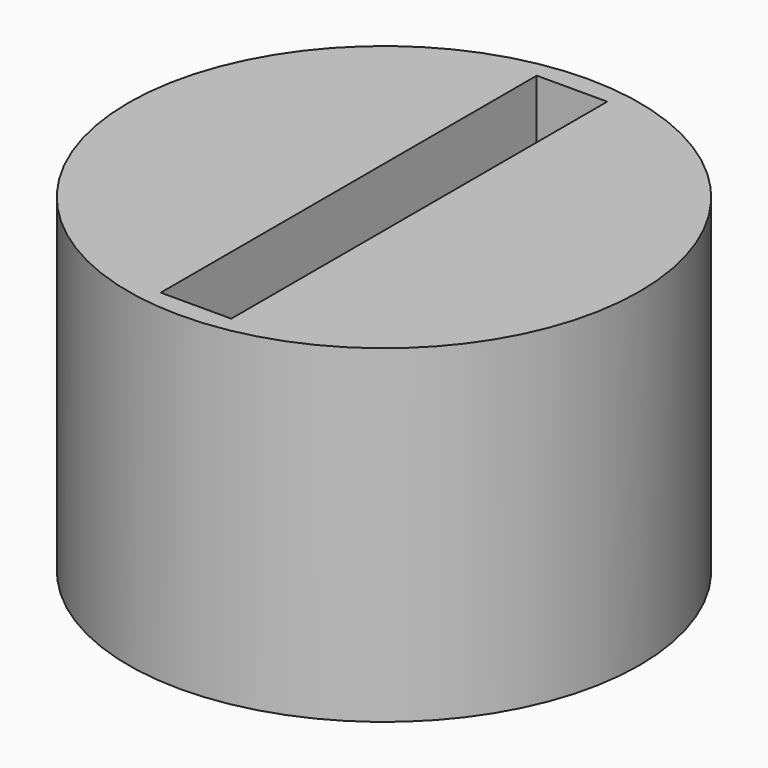
from build123d import *

# Parameters (mm, degrees)
F1_DEPTH        = 10
F2_R            = 21.75
F2_R_2          = 18.75
F3_DEPTH        = 20
F4_DEPTH        = 8
F7_DEPTH        = 3
F8_W            = 6
F8_H            = 40
F9_DEPTH        = 5
F11_D           = 2.2
F11_CSINK_D     = 5.1
F11_CSINK_ANGLE = 90


# Not quite as in the source:
# - a pattern or mirror of a feature is missing from the dataset's text; its kind, count and spacing are read off the source's solid


with BuildPart() as f1:
    # F0 (on Top) → F1 (new body)
    with BuildSketch(Plane.XY):
        Polygon((6.8993357168, 11.95), (-6.8993357168, 11.95), (-13.7986714336, 0), (-6.8993357168, -11.95), (6.8993357168, -11.95), (13.7986714336, 0), align=None)
        Polygon((-10.3345698185, 0), (-5.1672849092, 8.95), (5.1672849092, 8.95), (10.3345698185, 0), (5.1672849092, -8.95), (-5.1672849092, -8.95), align=None, mode=Mode.SUBTRACT)
    extrude(amount=F1_DEPTH)



with BuildPart() as f3:
    # F2 (on face) → F3 (new body)
    with BuildSketch(Plane.XY.offset(10)):
        Circle(F2_R)
        Circle(F2_R_2, mode=Mode.SUBTRACT)
    extrude(amount=-F3_DEPTH)


with BuildPart() as f4:
    # F2 (on face) → F4 (new body)
    with BuildSketch(Plane.XY.offset(10)):
        Circle(F2_R)
        Circle(F2_R_2, mode=Mode.SUBTRACT)
        Circle(F2_R_2)
        Polygon((6.8993357168, 11.95), (13.7986714336, 0), (6.8993357168, -11.95), (-6.8993357168, -11.95), (-13.7986714336, 0), (-6.8993357168, 11.95), align=None, mode=Mode.SUBTRACT)
        Polygon((6.8993357168, -11.95), (13.7986714336, 0), (6.8993357168, 11.95), (-6.8993357168, 11.95), (-13.7986714336, 0), (-6.8993357168, -11.95), align=None)
        Polygon((5.1672849092, -8.95), (-5.1672849092, -8.95), (-10.3345698185, 0), (-5.1672849092, 8.95), (5.1672849092, 8.95), (10.3345698185, 0), align=None, mode=Mode.SUBTRACT)
        Polygon((-10.3345698185, 0), (-5.1672849092, -8.95), (5.1672849092, -8.95), (10.3345698185, 0), (5.1672849092, 8.95), (-5.1672849092, 8.95), align=None)
    extrude(amount=F4_DEPTH)


with BuildPart() as f1_1:
    add(f1.part)

    add(f3.part)  # F7 merges F3

    add(f4.part)  # F7 merges F4
    # F6 (on face) → F7 (join)
    with BuildSketch(Plane(origin=(5.3550892957, 3.0917622464, -5.9713601914), x_dir=(0.7822484827, -0.2864336826, 0.5532115841), z_dir=(0.622966541, 0.3596699002, -0.6946583705))):
        Polygon((7.5026214932, -3.9601203317), (5.2654806886, -6.6518114397), (15.9953805493, -15.5697354674), (18.2325213539, -12.8780443594), align=None)
    f7 = extrude(amount=-F7_DEPTH)

    # F7_copies: F7 across plane
    add(f7.mirror(Plane(origin=(0, 0, 0), x_dir=(0, 0, -1), z_dir=(0, -1, 0))))

    # F7_copies1: F7 across plane
    add(f7.mirror(Plane(origin=(0, 0, 0), x_dir=(0, 0, -1), z_dir=(-1, 0, 0))))

    # F7_copies2: F7 across plane
    add(f7.mirror(Plane(origin=(0, 0, 0), x_dir=(0.5, -0.8660254038, 0), z_dir=(-0.8660254038, -0.5, 0))))

    # F8 (on face) → F9 (cut)
    with BuildSketch(Plane.XY.offset(18)):
        Rectangle(F8_W, F8_H)
    extrude(amount=-F9_DEPTH, mode=Mode.SUBTRACT)

    # F11 (through all)
    with Locations(Plane(origin=(0, 0, 10), x_dir=(1, 0, 0), z_dir=(0, 0, -1))):
        with Locations((0, 15), (0, -15)):
            CounterSinkHole(F11_D / 2, F11_CSINK_D / 2, counter_sink_angle=F11_CSINK_ANGLE)


solid = f1_1.part
